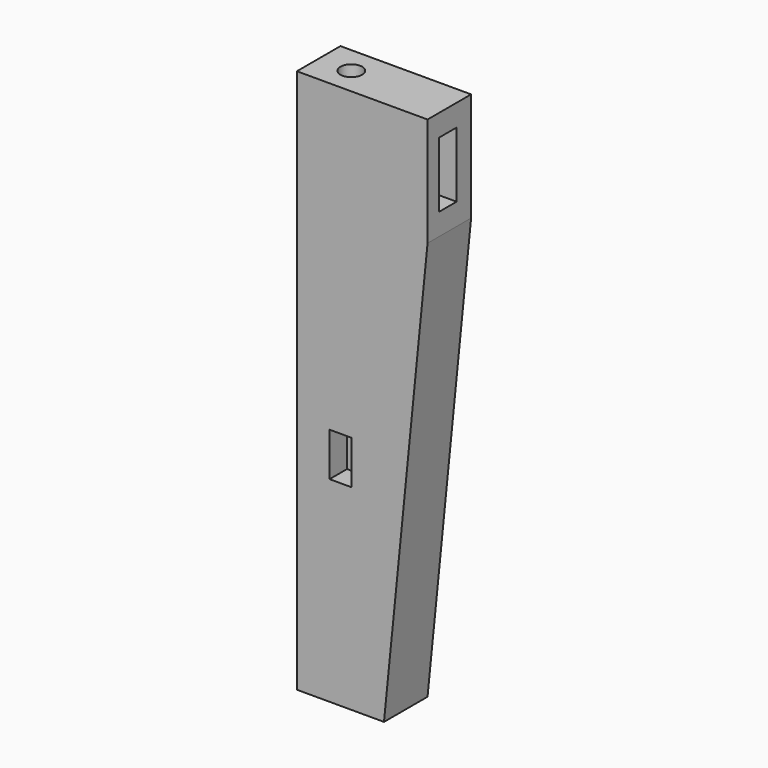
from build123d import *

# Parameters (mm, degrees)
F1_DEPTH = 25
F2_W     = 10
F2_H     = 20
F3_DEPTH = 10
F4_W     = 10
F4_H     = 30
F5_DEPTH = 25
F6_R     = 5
F7_DEPTH = 25


# Not quite as in the source:
# - a feature names something its author has since deleted; it is built from what else it names


with BuildPart() as f1:
    # F0 (on Front) → F1 (new body)
    with BuildSketch(Plane.XZ):
        Polygon((30, 186.9314253517), (-30, 186.9314253517), (-30, -63.0685746483), (10, -63.0685746483), (30, 136.9314253517), align=None)
    extrude(amount=F1_DEPTH)

    # F2 (on face) → F3 (cut)
    with BuildSketch(Plane.XZ.offset(25)):
        with Locations((-10, 36.9314253517)):
            Rectangle(F2_W, F2_H)
    extrude(amount=-F3_DEPTH, mode=Mode.SUBTRACT)

    # F4 (on face) → F5 (cut)
    with BuildSketch(Plane.YZ.offset(30)):
        with Locations((-13.3319108949, 161.9314253517)):
            Rectangle(F4_W, F4_H)
    extrude(amount=-F5_DEPTH, mode=Mode.SUBTRACT)

    # F6 (on face) → F7 (cut)
    with BuildSketch(Plane.XY.offset(186.9314253517)):
        with Locations((-15, -12.5)):
            Circle(F6_R)
    extrude(amount=-F7_DEPTH, mode=Mode.SUBTRACT)


solid = f1.part
